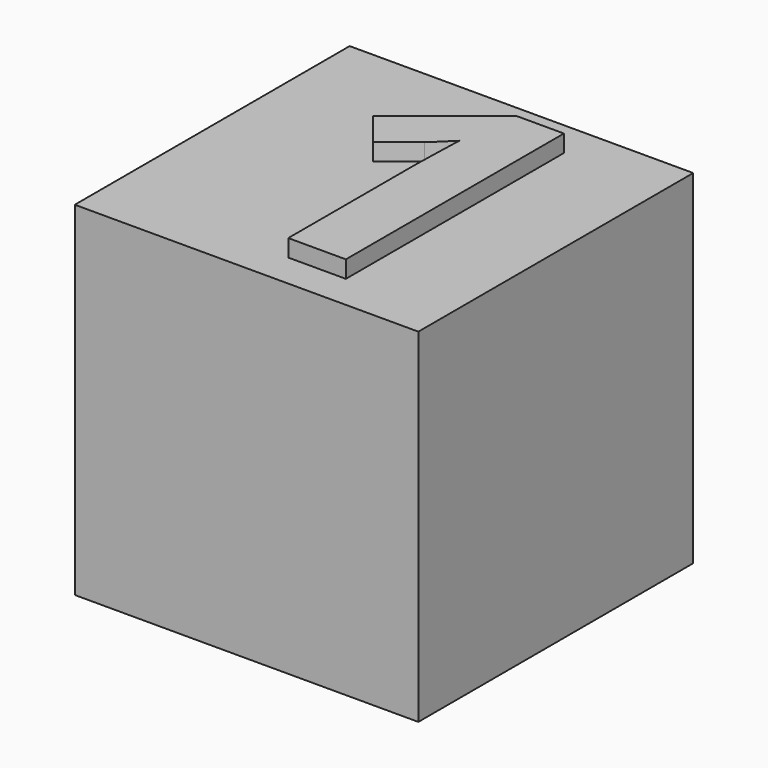
from build123d import *

# Parameters (mm, degrees)
F0_W         = 10
F0_H         = 10
F1_DEPTH     = 10
F2_TEXT_SIZE = 11.1111111111
F3_DEPTH     = 0.5


# Not quite as in the source:
# - Text() gives the source's letters only with a copy of the font that has no kerning and outlines rounded to 1/6400 em; it was checked with that copy


with BuildPart() as f1:
    # F0 (on Top) → F1 (new body)
    with BuildSketch(Plane.XY):
        with Locations((5, 5)):
            Rectangle(F0_W, F0_H)
    extrude(amount=F1_DEPTH)

    # F2 (on face) → F3 (join)
    with BuildSketch(Plane.XY.offset(10)):
        with Locations((2.5, 1)):
            Text('1', F2_TEXT_SIZE, font='Open Sans', font_style=FontStyle.BOLD, text_align=(TextAlign.LEFT, TextAlign.BOTTOM))
    extrude(amount=F3_DEPTH)


solid = f1.part
